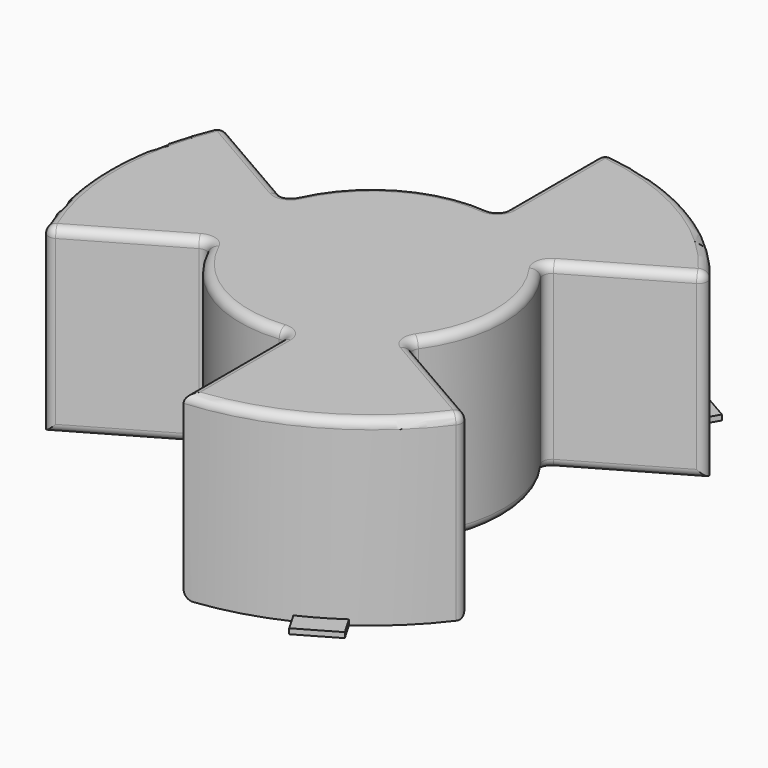
from build123d import *

# Parameters (mm, degrees)
F0_R     = 38.1
F1_DEPTH = 52.324
F3_DEPTH = 52.324
F4_W     = 6.35
F4_H     = 12.7
F5_DEPTH = 1.524
F6_R     = 2.54


with BuildPart() as f1:
    # F0 (on Top) → F1 (new body)
    with BuildSketch(Plane.XY):
        Circle(F0_R)
    extrude(amount=F1_DEPTH)

    # F2 (on Top) → F3 (join, through all)
    with BuildSketch(Plane.XY):
        with BuildLine():
            Line((6.35, -37.5671066227), (6.35, -75.9349557187))
            ThreePointArc((6.35, -75.9349557187), (38.1000001588, -65.9911356767), (62.5866008968, -43.4667388722))
            Line((62.5866008968, -43.4667388722), (29.3590689181, -24.2828143398))
            ThreePointArc((29.3590689181, -24.2828143398), (19.0500001605, -32.9955677915), (6.35, -37.5671066227))
        make_face()
        with BuildLine():
            ThreePointArc((6.3499996346, 37.5671066844), (19.0499998395, 32.9955679768), (29.3590686819, 24.2828146254))
            Line((29.3590686819, 24.2828146254), (62.5866006876, 43.4667391734))
            ThreePointArc((62.5866006876, 43.4667391734), (38.0999998412, 65.99113586), (6.3499996346, 75.9349557492))
            Line((6.3499996346, 75.9349557492), (6.3499996346, 37.5671066844))
        make_face()
        with BuildLine():
            ThreePointArc((-35.7090685527, -13.2842923446), (-38.1, -1.853e-07), (-35.7090686819, 13.2842919973))
            Line((-35.7090686819, 13.2842919973), (-68.9366006876, 32.4682165453))
            ThreePointArc((-68.9366006876, 32.4682165453), (-76.2, -1.833e-07), (-68.9366005314, -32.468216877))
            Line((-68.9366005314, -32.468216877), (-35.7090685527, -13.2842923446))
        make_face()
    extrude(amount=F3_DEPTH)

    # F4 (on face) → F5 (join)
    with BuildSketch(Plane(origin=(0, 0, 0), x_dir=(1, 0, 0), z_dir=(0, 0, -1))):
        with Locations((-79.1099557187, 0)):
            Rectangle(F4_W, F4_H)
        Polygon((43.4667391734, -62.5866006876), (32.4682165453, -68.9366006876), (35.6432165453, -74.4358620017), (46.6417391734, -68.0858620017), align=None)
        Polygon((32.4682165453, 68.9366006876), (43.4667391734, 62.5866006876), (46.6417391734, 68.0858620017), (35.6432165453, 74.4358620017), align=None)
    extrude(amount=-F5_DEPTH)

    # F6
    f6_edges = [f1.edges().sort_by_distance(p)[0] for p in [
        (38.1, 0, 52.324),
        (45.972835, 33.874777, 52.324),
        (38.1, 65.991136, 52.324),
        (6.35, 56.751031, 52.324),
        (-19.05, 32.995568, 52.324),
        (-52.322835, 22.876254, 52.324),
        (-76.2, 0, 52.324),
        (-52.322835, -22.876255, 52.324),
        (-19.05, -32.995568, 52.324),
        (6.35, -56.751031, 52.324),
        (38.1, -65.991136, 52.324),
        (45.972835, -33.874777, 52.324),
        (6.35, -37.567107, 26.162),
        (-35.709069, -13.284292, 26.162),
        (-19.05, -32.995568, 0),
        (-68.936601, -32.468217, 26.162),
        (-19.05, 32.995568, 0),
        (-35.709069, 13.284292, 26.162),
        (6.35, 37.567107, 26.162),
        (-68.936601, 32.468217, 26.162),
        (6.35, 75.934956, 26.162),
        (38.1, 0, 0),
        (29.359069, -24.282814, 26.162),
        (29.359069, 24.282815, 26.162),
        (62.586601, 43.466739, 26.162),
        (62.586601, -43.466739, 26.162),
        (45.972835, 33.874777, 0),
        (6.35, 56.751031, 0),
        (-52.322835, 22.876254, 0),
        (-52.322835, -22.876255, 0),
        (6.35, -56.751031, 0),
        (45.972835, -33.874777, 0),
    ]]
    fillet(f6_edges, radius=F6_R)


solid = f1.part
